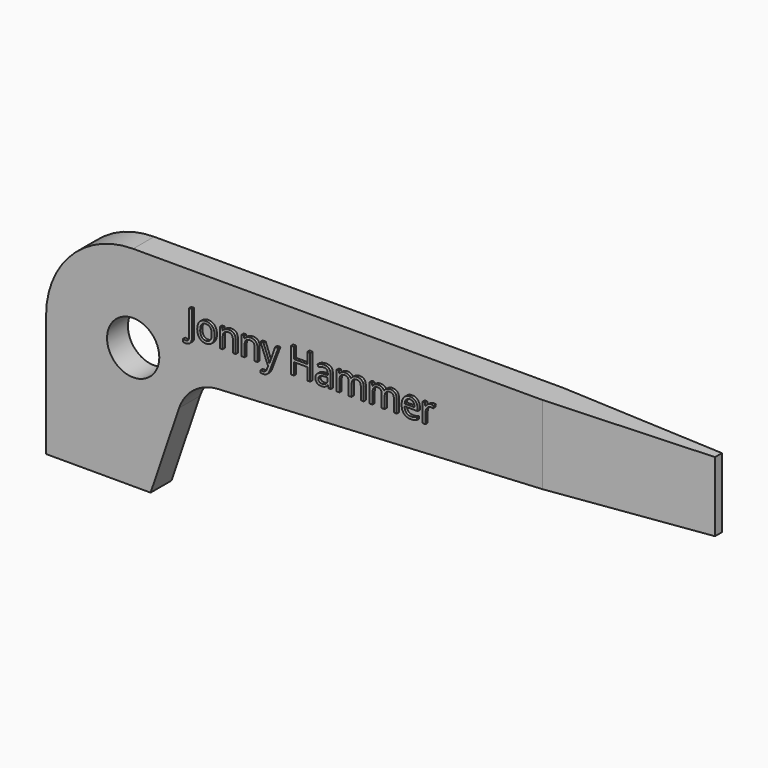
from build123d import *

# Parameters (mm, degrees)
F1_DEPTH     = 2.38125
F2_R         = 2.38125
F3_DEPTH     = 25.4
F5_DEPTH     = 25.4
F6_TEXT_SIZE = 3.2396210978
F7_DEPTH     = 0.254


# Not quite as in the source:
# - Text() gives the source's letters only with a copy of the font that has no kerning and outlines rounded to 1/6400 em; it was checked with that copy


with BuildPart() as f1:
    # F0 (on Front) → F1 (new body)
    with BuildSketch(Plane.XZ):
        with BuildLine():
            Line((60.325, 19.05), (7.9375, 19.05))
            ThreePointArc((7.9375, 19.05), (2.3248399243, 16.7251600757), (0, 11.1125))
            Line((0, 11.1125), (0, 0))
            Line((0, 0), (9.525, 0))
            Line((9.525, 0), (12.1173647876, 7.6271664624))
            ThreePointArc((12.1173647876, 7.6271664624), (13.4786145605, 9.5135918491), (15.6631963617, 10.3130942181))
            Line((15.6631963617, 10.3130942181), (60.325, 12.7))
            Line((60.325, 12.7), (60.325, 19.05))
        make_face()
    extrude(amount=F1_DEPTH)

    # F2 (on face) → F3 (cut)
    with BuildSketch(Plane.XZ.offset(2.38125)):
        with Locations((7.9375, 11.1125)):
            Circle(F2_R)
    extrude(amount=-F3_DEPTH, mode=Mode.SUBTRACT)

    # F4 (on face) → F5 (cut)
    with BuildSketch(Plane.XY.offset(19.05)):
        Polygon((60.325, -2.38125), (60.325, -1.5875), (45.2374, -2.38125), align=None)
        Polygon((60.325, 0), (45.2374, 0), (60.325, -0.79375), align=None)
    extrude(amount=-F5_DEPTH, mode=Mode.SUBTRACT)

    # F6 (on face) → F7 (join)
    with BuildSketch(Plane.XZ.offset(2.38125)):
        with Locations((12.9320919514, 13.8053633273)):
            Text('Jonny Hammer', F6_TEXT_SIZE, font='Open Sans', text_align=(TextAlign.LEFT, TextAlign.BOTTOM))
    extrude(amount=F7_DEPTH)


solid = f1.part
